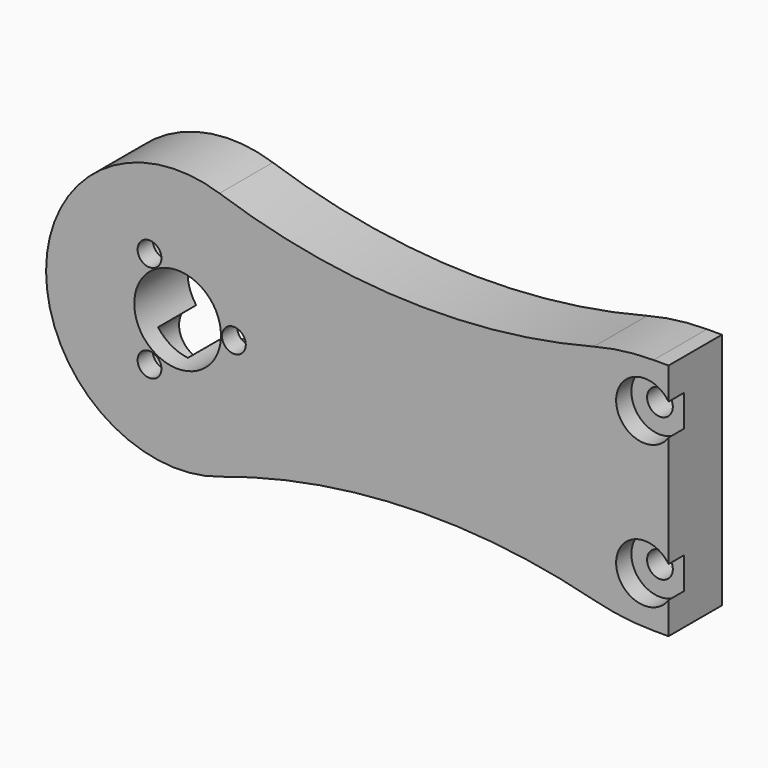
from build123d import *

# Parameters (mm, degrees)
F0_R           = 4.55
F1_DEPTH       = 7
F3_D           = 2.5
F3_CBORE_D     = 5
F3_CBORE_DEPTH = 5
F4_D           = 2.7
F4_CBORE_D     = 6
F4_CBORE_DEPTH = 2
F5_R           = 25


with BuildPart() as f1:
    # F0 (on Front) → F1 (new body)
    with BuildSketch(Plane.XZ):
        with BuildLine():
            ThreePointArc((4.3861063064, -13.0844209451), (11.2019700729, -8.0595202392), (13.8, 0))
            ThreePointArc((13.8, 0), (11.2019700729, 8.0595202392), (4.3861063064, 13.0844209451))
            ThreePointArc((4.3861063064, 13.0844209451), (-13.8, 0), (4.3861063064, -13.0844209451))
        make_face()
        Circle(F0_R, mode=Mode.SUBTRACT)
        with BuildLine():
            ThreePointArc((4.3861063064, 13.0844209451), (11.2019700729, 8.0595202392), (13.8, 0))
            ThreePointArc((13.8, 0), (11.2019700729, -8.0595202392), (4.3861063064, -13.0844209451))
            ThreePointArc((4.3861063064, -13.0844209451), (25.3974589974, -9.5066550069), (46.5, -12.5))
            Line((46.5, -12.5), (51.5, -12.5))
            Line((51.5, -12.5), (51.5, 12.5))
            Line((51.5, 12.5), (46.5, 12.5))
            ThreePointArc((46.5, 12.5), (25.3974589974, 9.5066550069), (4.3861063064, 13.0844209451))
        make_face()
    extrude(amount=F1_DEPTH)

    # F3 (through all)
    with Locations(Plane(origin=(0, 0, 0), x_dir=(1, 0, 0), z_dir=(0, 1, 0))):
        with Locations((-2.95, -5.1095498823), (-2.95, 5.1095498823), (5.9, 0)):
            CounterBoreHole(F3_D / 2, F3_CBORE_D / 2, F3_CBORE_DEPTH)

    # F4 (through all)
    with Locations(Plane.XZ.offset(7)):
        with Locations((49, 7.5), (49, -7.5)):
            CounterBoreHole(F4_D / 2, F4_CBORE_D / 2, F4_CBORE_DEPTH)

    # F5
    f5_edges = [f1.edges().sort_by_distance(p)[0] for p in [
        (46.5, -3.5, 12.5),
        (46.5, -3.5, -12.5),
    ]]
    fillet(f5_edges, radius=F5_R)


solid = f1.part
